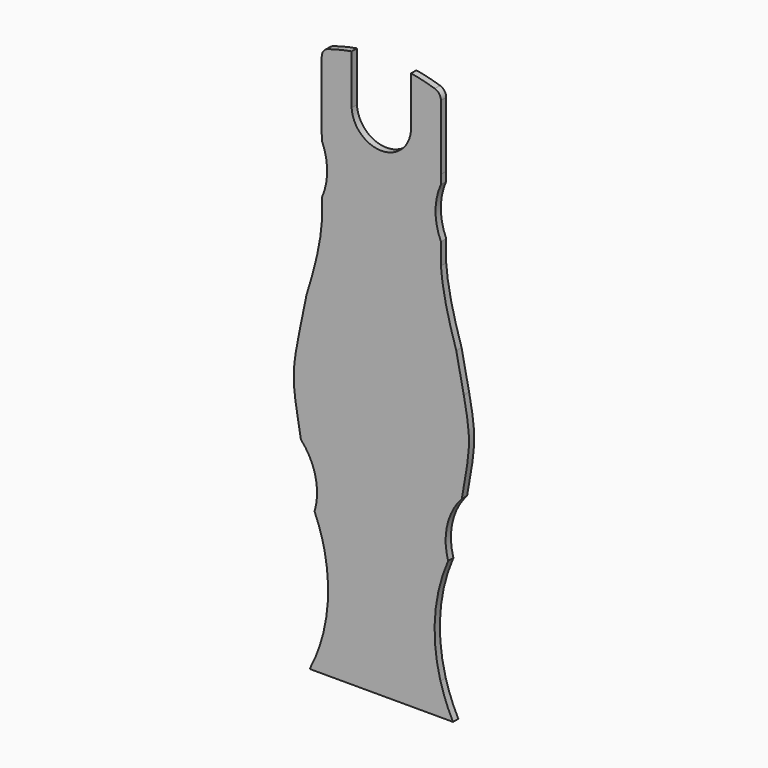
from build123d import *

# Parameters (mm, degrees)
F1_DEPTH = 3


with BuildPart() as f1:
    # F0 (on Front) → F1 (new body)
    with BuildSketch(Plane.XZ):
        with BuildLine():
            Line((-27.000000372, 67.3308055204), (-27.0000003572, 60.5094830675))
            add(Edge.make_bspline(
                [(-27.0000003783, 70.2132413448), (-27.000000372, 67.3308055204), (-26.8073760372, 64.0094927256), (-27.0000003572, 60.5094830675)],
                knots=[0, 0, 0, 0, 0.0797949898, 0.0797949898, 0.0797949898, 0.0797949898], degree=3))
            Line((-27.0000003783, 70.2132413448), (-27.000000372, 67.3308055204))
        make_face()
        with BuildLine():
            add(Edge.make_bspline(
                [(-27.0000003783, 70.2132413448), (-27.000000372, 67.3308055204), (-26.8073760372, 64.0094927256), (-27.0000003572, 60.5094830675)],
                knots=[0, 0, 0, 0, 0.0797949898, 0.0797949898, 0.0797949898, 0.0797949898], degree=3))
            add(Edge.make_bspline(
                [(-27.0000003572, 60.5094830675), (-27.2115741289, 56.665159338), (-28.5032848349, 48.9114242757), (-30.7959376047, 39.269131214), (-32.7990054786, 33.0934715655), (-33.9583066177, 28.9822912379)],
                knots=[0.0797949898, 0.0797949898, 0.0797949898, 0.0797949898, 0.1674398258, 0.2471817217, 0.3319487208, 0.3319487208, 0.3319487208, 0.3319487208], degree=3))
            add(Edge.make_bspline(
                [(-37.2038997366, 13.1717467116), (-36.2347795039, 17.9824819127), (-35.0866971891, 23.3074594843), (-33.9583066177, 28.9822912379)],
                knots=[0.7969356306, 0.7969356306, 0.7969356306, 0.7969356306, 1, 1, 1, 1], degree=3))
            add(Edge.make_bspline(
                [(-37.2038997366, 13.1717467116), (-37.3377860295, 11.7966552771), (-37.8318020205, 3.6131566189), (-34.8319401075, -9.4971781129), (-33.3481357614, -22.2384102756), (-27.0171200398, -42.5814503212), (-25.8644027957, -62.9931088525), (-25.7257572716, -70.2838279012)],
                knots=[0.4247645948, 0.4247645948, 0.4247645948, 0.4247645948, 0.4471809961, 0.5577287405, 0.6473745734, 0.7857235681, 0.8551599855, 0.8551599855, 0.8551599855, 0.8551599855], degree=3))
            ThreePointArc((-25.7257572716, -70.2838279012), (-24.1356221819, -86.7785971976), (-26.2738365605, -103.2113079605))
            add(Edge.make_bspline(
                [(-26.2738365605, -103.2113079605), (-26.4866600906, -108.6415730769), (-26.7346990947, -114.1409528022), (-26.9831408055, -119.6440920773)],
                knots=[0.952812329, 0.952812329, 0.952812329, 0.952812329, 0.9989562439, 0.9989562439, 0.9989562439, 0.9989562439], degree=3))
            Line((-26.9831408055, -119.6440920773), (0, -119.6440920773))
            Line((-6.3e-09, -119.6440920772), (26.9834561434, -119.6440920746))
            add(Edge.make_bspline(
                [(26.7797560592, -105.146393671), (26.7183865925, -110.0484100554), (26.7770637598, -114.8950679943), (26.9834561434, -119.6440920746)],
                knots=[0.9591803486, 0.9591803486, 0.9591803486, 0.9591803486, 0.9989568231, 0.9989568231, 0.9989568231, 0.9989568231], degree=3))
            ThreePointArc((26.7797560592, -105.146393671), (24.3110117736, -80.3279975292), (30.2677449554, -56.1088973147))
            ThreePointArc((30.2677449554, -56.1088973147), (29.3582502263, -44.7091117977), (33.0959109358, -33.901143306))
            add(Edge.make_bspline(
                [(37.3760657429, 12.312352727), (37.4207370145, 11.2848759506), (37.6386418394, 0.6550807977), (35.3777267818, -16.2805465578), (33.0959109358, -33.901143306)],
                knots=[0.5873705512, 0.5873705512, 0.5873705512, 0.5873705512, 0.6053891461, 0.7637611434, 0.7637611434, 0.7637611434, 0.7637611434], degree=3))
            add(Edge.make_bspline(
                [(37.3760657429, 12.312352727), (36.3723917785, 17.3454447873), (35.1543287191, 22.9673311954), (33.9583066177, 28.9822912379)],
                knots=[0.7847647083, 0.7847647083, 0.7847647083, 0.7847647083, 1, 1, 1, 1], degree=3))
            add(Edge.make_bspline(
                [(27.0000003572, 60.5094830675), (27.211196853, 56.9686043212), (28.5006041901, 48.7178368751), (30.8051136621, 39.5194264195), (32.7778690192, 32.6057451698), (33.9583066177, 28.9822912379)],
                knots=[0.1080256566, 0.1080256566, 0.1080256566, 0.1080256566, 0.2266783563, 0.3346321349, 0.449388848, 0.449388848, 0.449388848, 0.449388848], degree=3))
            add(Edge.make_bspline(
                [(27.0000003783, 70.2132413448), (27.0000003698, 66.3110286441), (26.8077195227, 63.7332255726), (27.0000003572, 60.5094830675)],
                knots=[0, 0, 0, 0, 0.1080256566, 0.1080256566, 0.1080256566, 0.1080256566], degree=3))
            ThreePointArc((27.0000003783, 70.2132413448), (24.5597225455, 81.642003215), (27.0140844765, 93.0677487616))
            Line((27.0140844765, 93.0677487616), (27.0165528594, 97.073236044))
            Line((27.0165528594, 97.073236044), (27.0165528594, 126.5655265976))
            ThreePointArc((27.0165528594, 126.5655265976), (26.2369988642, 128.9421564287), (24.1982364647, 130.3911290521))
            ThreePointArc((24.1982364647, 130.3911290521), (18.8821286754, 131.8789775648), (13.4760826795, 132.9967261563))
            Line((13.4760826795, 132.9967261563), (13.4760826795, 111.3308812648))
            ThreePointArc((13.4760826795, 111.3308812648), (0.4287985626, 97.7135570783), (-13.4581639711, 110.4734713575))
            ThreePointArc((-13.4581639711, 110.4734713575), (-13.4768872509, 111.1836209893), (-13.4581639711, 111.8937706212))
            Line((-13.4581639711, 111.8937706212), (-13.4581639711, 132.9915701483))
            ThreePointArc((-13.4581639711, 132.9915701483), (-18.8878136613, 131.8714457801), (-24.2268647008, 130.3780240861))
            ThreePointArc((-24.2268647008, 130.3780240861), (-26.2446496183, 128.9275955182), (-27.0165494938, 126.5655265976))
            Line((-27.0165494938, 126.5655265976), (-27.0165494938, 97.073236044))
            Line((-27.0165494938, 97.073236044), (-27.0094336483, 93.0702374443))
            ThreePointArc((-27.0094336483, 93.0702374443), (-24.5568387649, 81.642749654), (-27.0000003783, 70.2132413448))
        make_face()
        with BuildLine():
            add(Edge.make_bspline(
                [(-37.2038997366, 13.1717467116), (-37.3377860295, 11.7966552771), (-37.8318020205, 3.6131566189), (-34.8319401075, -9.4971781129), (-33.3481357614, -22.2384102756), (-27.0171200398, -42.5814503212), (-25.8644027957, -62.9931088525), (-25.7257572716, -70.2838279012)],
                knots=[0.4247645948, 0.4247645948, 0.4247645948, 0.4247645948, 0.4471809961, 0.5577287405, 0.6473745734, 0.7857235681, 0.8551599855, 0.8551599855, 0.8551599855, 0.8551599855], degree=3))
            add(Edge.make_bspline(
                [(-36.4695142582, -29.3788072578), (-37.5997978701, -23.1616359537), (-39.5544950983, -12.3662754957), (-40.0648496415, -1.9518214908), (-38.2132158377, 8.1614782915), (-37.2038997366, 13.1717467116)],
                knots=[0, 0, 0, 0, 0.3165678715, 0.5854488298, 0.7969356306, 0.7969356306, 0.7969356306, 0.7969356306], degree=3))
            ThreePointArc((-36.4695142582, -29.3788072578), (-29.8578197059, -41.9292933744), (-30.2677449554, -56.1088973147))
            ThreePointArc((-30.2677449554, -56.1088973147), (-27.6377010863, -63.081314369), (-25.7257572716, -70.2838279012))
        make_face()
        with BuildLine():
            add(Edge.make_bspline(
                [(-26.2738365605, -103.2113079605), (-26.4866600906, -108.6415730769), (-26.7346990947, -114.1409528022), (-26.9831408055, -119.6440920773)],
                knots=[0.952812329, 0.952812329, 0.952812329, 0.952812329, 0.9989562439, 0.9989562439, 0.9989562439, 0.9989562439], degree=3))
            ThreePointArc((-26.2738365605, -103.2113079605), (-28.8907910345, -111.6137859631), (-32.4913841825, -119.6440920773))
            Line((-32.4913841825, -119.6440920773), (-26.9831408055, -119.6440920773))
        make_face()
        with BuildLine():
            Line((-13.4581639711, 110.4734713575), (-13.4581639711, 111.8937706212))
            ThreePointArc((-13.4581639711, 111.8937706212), (-13.4768872509, 111.1836209893), (-13.4581639711, 110.4734713575))
        make_face()
        with BuildLine():
            add(Edge.make_bspline(
                [(26.7797560592, -105.146393671), (26.7183865925, -110.0484100554), (26.7770637598, -114.8950679943), (26.9834561434, -119.6440920746)],
                knots=[0.9591803486, 0.9591803486, 0.9591803486, 0.9591803486, 0.9989568231, 0.9989568231, 0.9989568231, 0.9989568231], degree=3))
            Line((26.9834561434, -119.6440920746), (32.4913842119, -119.644092074))
            ThreePointArc((32.4913841825, -119.6440920773), (29.2510439227, -112.5467338616), (26.7797560592, -105.146393671))
        make_face()
        with BuildLine():
            add(Edge.make_bspline(
                [(37.3760657429, 12.312352727), (37.4207370145, 11.2848759506), (37.6386418394, 0.6550807977), (35.3777267818, -16.2805465578), (33.0959109358, -33.901143306)],
                knots=[0.5873705512, 0.5873705512, 0.5873705512, 0.5873705512, 0.6053891461, 0.7637611434, 0.7637611434, 0.7637611434, 0.7637611434], degree=3))
            ThreePointArc((33.0959109358, -33.901143306), (34.6666972167, -31.5542800935), (36.4665470243, -29.37811899))
            add(Edge.make_bspline(
                [(36.4665470243, -29.37811899), (37.596826169, -23.1609722577), (39.5556506505, -12.3664838808), (40.0569196281, -2.1108359245), (38.3055086703, 7.651504698), (37.3760657429, 12.312352727)],
                knots=[0, 0, 0, 0, 0.3165666204, 0.5854480709, 0.7847647083, 0.7847647083, 0.7847647083, 0.7847647083], degree=3))
        make_face()
        with BuildLine():
            add(Edge.make_bspline(
                [(27.0000003783, 70.2132413448), (27.0000003698, 66.3110286441), (26.8077195227, 63.7332255726), (27.0000003572, 60.5094830675)],
                knots=[0, 0, 0, 0, 0.1080256566, 0.1080256566, 0.1080256566, 0.1080256566], degree=3))
            Line((27.0000003572, 60.5094830675), (27.0000003783, 70.2132413448))
        make_face()
    extrude(amount=F1_DEPTH)


solid = f1.part
